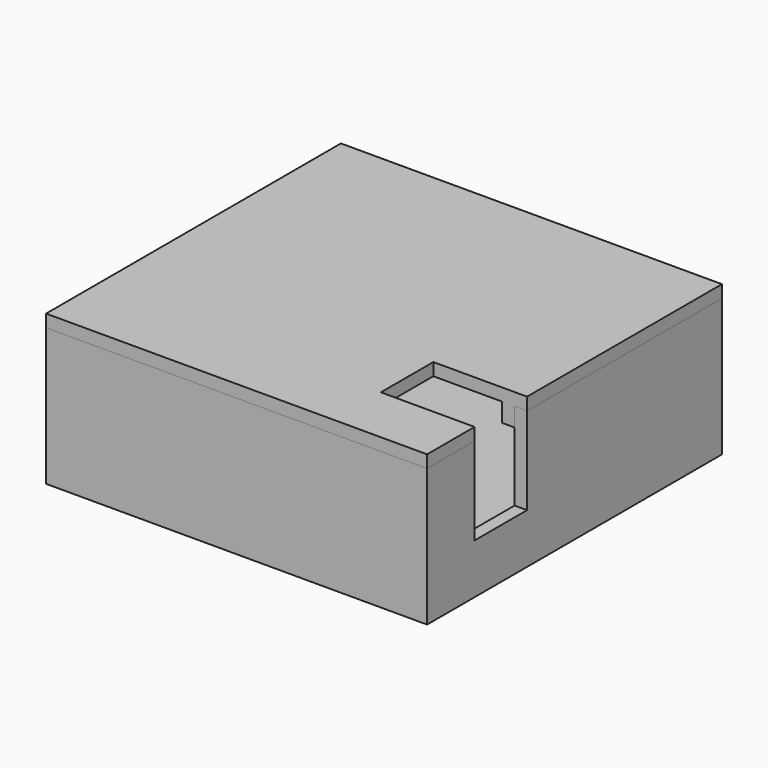
from build123d import *

# Parameters (mm, degrees)
F1_DEPTH  = 2
F2_DEPTH  = 20
F4_W      = 31
F4_H      = 14
F5_DEPTH  = 2
F7_W      = 10.5
F7_H      = 14
F8_DEPTH  = 2
F4_W_2    = 9.6
F4_H_2    = 5.9
F9_DEPTH  = 25
F11_W     = 8
F11_H     = 30
F12_DEPTH = 2
F13_DEPTH = 3
F14_DEPTH = 3
F15_DEPTH = 4


with BuildPart() as f1:
    # F0 (on Top) → F1 (new body)
    with BuildSketch(Plane.XY):
        Polygon((-30.5, 29.5), (-30.5, -4.5), (-30.5, -29.5), (30.5, -29.5), (30.5, 29.5), align=None)
        Polygon((28.5, -23.5), (28.5, -27.5), (24.5, -27.5), (-24.5, -27.5), (-28.5, -27.5), (-28.5, -23.5), (-28.5, -4.5), (-28.5, 23.5), (-28.5, 27.5), (-24.5, 27.5), (24.5, 27.5), (28.5, 27.5), (28.5, 23.5), align=None, mode=Mode.SUBTRACT)
        Polygon((24.5, -27.5), (28.5, -27.5), (28.5, -23.5), (26.5, -23.5), (26.5, -25.5), (24.5, -25.5), align=None)
        Polygon((-24.5, -27.5), (24.5, -27.5), (24.5, -25.5), (26.5, -25.5), (26.5, -23.5), (28.5, -23.5), (28.5, 23.5), (26.5, 23.5), (26.5, 25.5), (24.5, 25.5), (24.5, 27.5), (-24.5, 27.5), (-24.5, 25.5), (-26.5, 25.5), (-26.5, 23.5), (-28.5, 23.5), (-28.5, -4.5), (-28.5, -23.5), (-26.5, -23.5), (-26.5, -25.5), (-24.5, -25.5), align=None)
        Polygon((-28.5, -27.5), (-24.5, -27.5), (-24.5, -25.5), (-26.5, -25.5), (-26.5, -23.5), (-28.5, -23.5), align=None)
        Polygon((26.5, 23.5), (28.5, 23.5), (28.5, 27.5), (24.5, 27.5), (24.5, 25.5), (26.5, 25.5), align=None)
        Polygon((-24.5, 25.5), (-24.5, 27.5), (-28.5, 27.5), (-28.5, 23.5), (-26.5, 23.5), (-26.5, 25.5), align=None)
    extrude(amount=-F1_DEPTH)

    # F0 (on Top) → F2 (join)
    with BuildSketch(Plane.XY):
        Polygon((-30.5, 29.5), (-30.5, -4.5), (-30.5, -29.5), (30.5, -29.5), (30.5, 29.5), align=None)
        Polygon((28.5, -23.5), (28.5, -27.5), (24.5, -27.5), (-24.5, -27.5), (-28.5, -27.5), (-28.5, -23.5), (-28.5, -4.5), (-28.5, 23.5), (-28.5, 27.5), (-24.5, 27.5), (24.5, 27.5), (28.5, 27.5), (28.5, 23.5), align=None, mode=Mode.SUBTRACT)
    extrude(amount=F2_DEPTH)

    # F4 (on offset) → F5 (cut, through all)
    with BuildSketch(Plane.YZ.offset(-30.5)):
        with Locations((11, 13)):
            Rectangle(F4_W, F4_H)
    extrude(amount=F5_DEPTH, mode=Mode.SUBTRACT)

    # F7 (on offset) → F8 (cut, through all)
    with BuildSketch(Plane.YZ.offset(30.5)):
        with Locations((-14.75, 13)):
            Rectangle(F7_W, F7_H)
    extrude(amount=-F8_DEPTH, mode=Mode.SUBTRACT)

    # F4 (on offset) → F9 (cut)
    with BuildSketch(Plane.YZ.offset(-30.5)):
        with Locations((-14, 13.9)):
            Rectangle(F4_W_2, F4_H_2)
    extrude(amount=F9_DEPTH, mode=Mode.SUBTRACT)

    # F0 (on Top) → F15 (join)
    with BuildSketch(Plane.XY):
        Polygon((26.5, 23.5), (28.5, 23.5), (28.5, 27.5), (24.5, 27.5), (24.5, 25.5), (26.5, 25.5), align=None)
        Polygon((-24.5, 25.5), (-24.5, 27.5), (-28.5, 27.5), (-28.5, 23.5), (-26.5, 23.5), (-26.5, 25.5), align=None)
        Polygon((-28.5, -27.5), (-24.5, -27.5), (-24.5, -25.5), (-26.5, -25.5), (-26.5, -23.5), (-28.5, -23.5), align=None)
        Polygon((24.5, -27.5), (28.5, -27.5), (28.5, -23.5), (26.5, -23.5), (26.5, -25.5), (24.5, -25.5), align=None)
    extrude(amount=F15_DEPTH)


with BuildPart() as f12:
    # F11 (on offset) → F12 (new body)
    with BuildSketch(Plane.XY.offset(20)):
        Polygon((28.5, -20), (28.5, -27.5), (-28.5, -27.5), (-28.5, -4.5), (-28.5, 27.5), (-18.5, 27.5), (28.5, 27.5), (28.5, -9.5), (30.5, -9.5), (30.5, 29.5), (-30.5, 29.5), (-30.5, -29.5), (30.5, -29.5), (30.5, -20), align=None)
        Polygon((26.5, -25.5), (26.5, -20), (15.5, -20), (15.5, -9.5), (26.5, -9.5), (26.5, 25.5), (-18.5, 25.5), (-18.5, -4.5), (-26.5, -4.5), (-26.5, -25.5), align=None)
        Polygon((-28.5, -27.5), (28.5, -27.5), (28.5, -20), (26.5, -20), (26.5, -25.5), (-26.5, -25.5), (-26.5, -4.5), (-28.5, -4.5), align=None)
        with Locations((-22.5, 10.5)):
            Rectangle(F11_W, F11_H)
        Polygon((-28.5, 27.5), (-28.5, -4.5), (-26.5, -4.5), (-26.5, 25.5), (-18.5, 25.5), (-18.5, 27.5), align=None)
        Polygon((26.5, -9.5), (28.5, -9.5), (28.5, 27.5), (-18.5, 27.5), (-18.5, 25.5), (26.5, 25.5), align=None)
    extrude(amount=F12_DEPTH)

    # F11 (on offset) → F13 (join)
    with BuildSketch(Plane.XY.offset(20)):
        Polygon((-28.5, -27.5), (28.5, -27.5), (28.5, -20), (26.5, -20), (26.5, -25.5), (-26.5, -25.5), (-26.5, -4.5), (-28.5, -4.5), align=None)
        Polygon((-28.5, 27.5), (-28.5, -4.5), (-26.5, -4.5), (-26.5, 25.5), (-18.5, 25.5), (-18.5, 27.5), align=None)
        Polygon((26.5, -9.5), (28.5, -9.5), (28.5, 27.5), (-18.5, 27.5), (-18.5, 25.5), (26.5, 25.5), align=None)
    extrude(amount=-F13_DEPTH)

    # F11 (on offset) → F14 (cut)
    with BuildSketch(Plane.XY.offset(20)):
        with Locations((-22.5, 10.5)):
            Rectangle(F11_W, F11_H)
        Polygon((-28.5, 27.5), (-28.5, -4.5), (-26.5, -4.5), (-26.5, 25.5), (-18.5, 25.5), (-18.5, 27.5), align=None)
    extrude(amount=-F14_DEPTH, mode=Mode.SUBTRACT)


solid = Compound([f1.part, f12.part])
